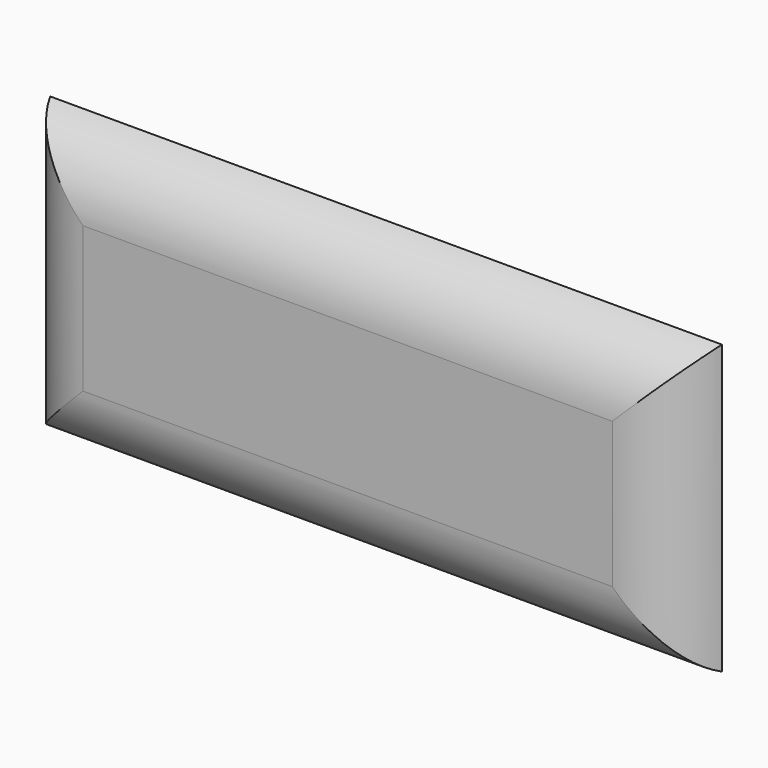
from build123d import *

# Parameters (mm, degrees)
F0_W        = 88.9
F0_H        = 6.35
F1_DEPTH    = 38.1
F2_T1_DEPTH = 135.9928603931
F2_T3_DEPTH = 85.1928603931


# Not quite as in the source:
# - a fillet or chamfer that OpenCascade refuses, or shapes differently, is made with other operations: its cross-section is extruded or revolved along the edge and cut away or added


with BuildPart() as f1:
    # F0 (on Top) → F1 (new body)
    with BuildSketch(Plane.XY):
        with Locations((-98.556979218, -8.8337444547)):
            Rectangle(F0_W, F0_H)
    extrude(amount=F1_DEPTH)

    # F2: fillet of radius 10.16 on 4 edges, made by hand

    # F2_s2 → F2_t1 (cut)
    with BuildSketch(Plane.YZ.offset(-166.5534094146)):
        with BuildLine():
            ThreePointArc((-12.0087444547, 28.6814279214), (-10.2729714222, 34.3610405842), (-5.6587444547, 38.1))
            Line((-5.6587444547, 38.1), (-12.0087444547, 38.1))
            Line((-12.0087444547, 38.1), (-12.0087444547, 28.6814279214))
        make_face()
        with BuildLine():
            ThreePointArc((-12.0087444547, 9.4185720786), (-10.2729714222, 3.7389594158), (-5.6587444547, 0))
            Line((-5.6587444547, 0), (-12.0087444547, 0))
            Line((-12.0087444547, 0), (-12.0087444547, 9.4185720786))
        make_face()
    extrude(amount=F2_T1_DEPTH, mode=Mode.SUBTRACT)

    # F2_s4 → F2_t3 (cut)
    with BuildSketch(Plane.XY.offset(-23.5464301965)):
        with BuildLine():
            ThreePointArc((-54.106979218, -5.6587444547), (-57.8459386338, -10.2729714222), (-63.5255512967, -12.0087444547))
            Line((-63.5255512967, -12.0087444547), (-54.106979218, -12.0087444547))
            Line((-54.106979218, -12.0087444547), (-54.106979218, -5.6587444547))
        make_face()
        with BuildLine():
            ThreePointArc((-143.006979218, -5.6587444547), (-139.2680198023, -10.2729714222), (-133.5884071394, -12.0087444547))
            Line((-133.5884071394, -12.0087444547), (-143.006979218, -12.0087444547))
            Line((-143.006979218, -12.0087444547), (-143.006979218, -5.6587444547))
        make_face()
    extrude(amount=F2_T3_DEPTH, mode=Mode.SUBTRACT)


solid = f1.part
